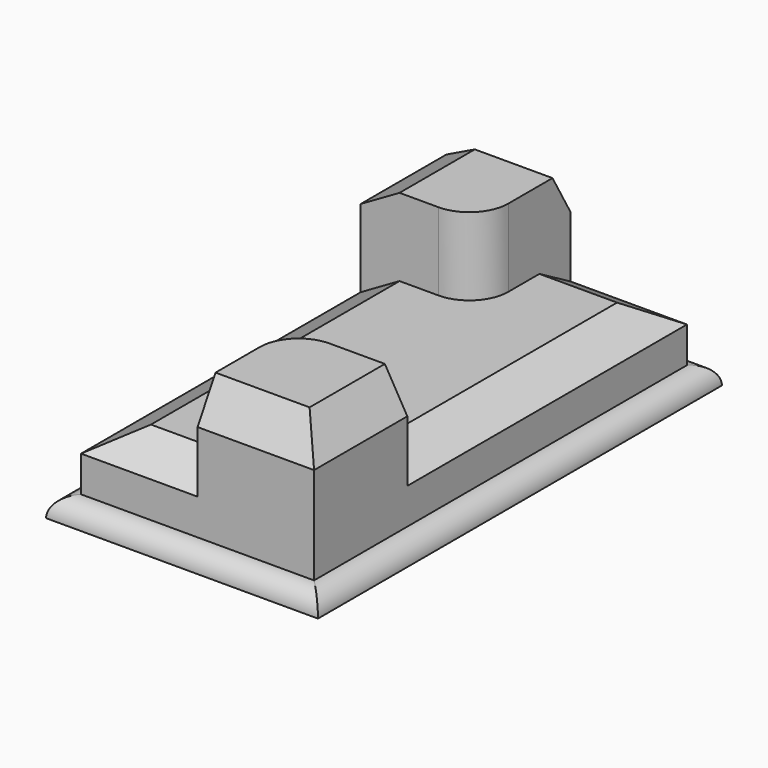
from build123d import *

# Parameters (mm, degrees)
F1_DEPTH    = 50.8
F2_DEPTH    = 25.4
F0_W        = 88.9
F0_H        = 165.1
F3_DEPTH    = 6.35
F4_SIZE2    = 7.3323484187
F4_SIZE     = 12.7
F5_C1_SIZE2 = 7.3323484187
F5_C1_SIZE  = 12.7
F5_C2_SIZE2 = 7.3323484187
F5_C2_SIZE  = 12.7
F5_C3_SIZE2 = 12.7
F5_C3_SIZE  = 7.3323484187
F5_C4_SIZE2 = 7.3323484187
F5_C4_SIZE  = 12.7
F6_R        = 6.34999


# Not quite as in the source:
# - a fillet or chamfer is up to 0.001 mm smaller than in the source, because OpenCascade refuses the exact size


with BuildPart() as f1:
    # F0 (on Top) → F1 (new body)
    with BuildSketch(Plane.XY):
        with BuildLine():
            Line((-19.9555572391, -85.2174787462), (-19.9555572391, -47.1174787462))
            Line((-19.9555572391, -47.1174787462), (-45.3555572391, -47.1174787462))
            ThreePointArc((-45.3555572391, -47.1174787462), (-54.3358133601, -50.8372226251), (-58.0555572391, -59.8174787462))
            Line((-58.0555572391, -59.8174787462), (-58.0555572391, -85.2174787462))
            Line((-58.0555572391, -85.2174787462), (-19.9555572391, -85.2174787462))
        make_face()
    extrude(amount=F1_DEPTH)



with BuildPart() as f1b:
    # F0 (on Top) → F1, piece 2 (new body)
    with BuildSketch(Plane.XY):
        with BuildLine():
            Line((-58.0555572391, 67.1825212538), (-96.1555572391, 67.1825212538))
            Line((-96.1555572391, 67.1825212538), (-96.1555572391, 29.0825212538))
            Line((-96.1555572391, 29.0825212538), (-70.7555572391, 29.0825212538))
            ThreePointArc((-70.7555572391, 29.0825212538), (-61.775301118, 32.8022651328), (-58.0555572391, 41.7825212538))
            Line((-58.0555572391, 41.7825212538), (-58.0555572391, 67.1825212538))
        make_face()
    extrude(amount=F1_DEPTH)


with BuildPart() as f1_1:
    add(f1.part)

    add(f1b.part)  # F2 merges F1b
    # F0 (on Top) → F2 (join)
    with BuildSketch(Plane.XY):
        with BuildLine():
            Line((-19.9555572391, 67.1825212538), (-58.0555572391, 67.1825212538))
            Line((-58.0555572391, 67.1825212538), (-58.0555572391, 41.7825212538))
            ThreePointArc((-58.0555572391, 41.7825212538), (-61.775301118, 32.8022651328), (-70.7555572391, 29.0825212538))
            Line((-70.7555572391, 29.0825212538), (-96.1555572391, 29.0825212538))
            Line((-96.1555572391, 29.0825212538), (-96.1555572391, -85.2174787462))
            Line((-96.1555572391, -85.2174787462), (-58.0555572391, -85.2174787462))
            Line((-58.0555572391, -85.2174787462), (-58.0555572391, -59.8174787462))
            ThreePointArc((-58.0555572391, -59.8174787462), (-54.3358133601, -50.8372226251), (-45.3555572391, -47.1174787462))
            Line((-45.3555572391, -47.1174787462), (-19.9555572391, -47.1174787462))
            Line((-19.9555572391, -47.1174787462), (-19.9555572391, 67.1825212538))
        make_face()
    extrude(amount=F2_DEPTH)

    # F0 (on Top) → F3 (join)
    with BuildSketch(Plane.XY):
        with Locations((-58.0555572391, -9.0174787462)):
            Rectangle(F0_W, F0_H)
        Polygon((-96.1555572391, 29.0825212538), (-96.1555572391, 67.1825212538), (-58.0555572391, 67.1825212538), (-19.9555572391, 67.1825212538), (-19.9555572391, -47.1174787462), (-19.9555572391, -85.2174787462), (-58.0555572391, -85.2174787462), (-96.1555572391, -85.2174787462), align=None, mode=Mode.SUBTRACT)
    extrude(amount=F3_DEPTH)

    # F4
    f4_edges = [f1_1.edges().sort_by_distance(p)[0] for p in [
        (-96.155557, -28.067479, 25.4),
        (-77.105557, -85.217479, 25.4),
        (-19.955557, 10.032521, 25.4),
        (-39.005557, 67.182521, 25.4),
    ]]
    f4_side = f1_1.faces().sort_by_distance((-58.055557, -9.017479, 25.4))[0]
    chamfer(f4_edges, length=F4_SIZE, length2=F4_SIZE2, reference=f4_side)

    # F5: chamfer of 12.7 x 7.3323484187 on 4 edges, made by hand

    # F5_c1
    f5_c1_edges = [f1_1.edges().sort_by_distance(p)[0] for p in [
        (-77.1055572391, 67.1825212538, 50.8),
    ]]
    f5_c1_side = f1_1.faces().sort_by_distance((-77.1055572391, 67.1825212538, 50.6533530316))[0]
    chamfer(f5_c1_edges, length=F5_C1_SIZE, length2=F5_C1_SIZE2, reference=f5_c1_side)

    # F5_c2
    f5_c2_edges = [f1_1.edges().sort_by_distance(p)[0] for p in [
        (-19.9555572391, -66.1674787462, 50.8),
    ]]
    f5_c2_side = f1_1.faces().sort_by_distance((-19.9555572391, -66.1674787462, 50.6533530316))[0]
    chamfer(f5_c2_edges, length=F5_C2_SIZE, length2=F5_C2_SIZE2, reference=f5_c2_side)

    # F5_c3
    f5_c3_edges = [f1_1.edges().sort_by_distance(p)[0] for p in [
        (-96.1555572391, 44.4663470445, 50.8),
    ]]
    f5_c3_side = f1_1.faces().sort_by_distance((-96.1555572391, 44.4663470445, 50.6533530316))[0]
    chamfer(f5_c3_edges, length=F5_C3_SIZE, length2=F5_C3_SIZE2, reference=f5_c3_side)

    # F5_c4
    f5_c4_edges = [f1_1.edges().sort_by_distance(p)[0] for p in [
        (-42.6717314484, -85.2174787462, 50.8),
    ]]
    f5_c4_side = f1_1.faces().sort_by_distance((-42.6717314484, -85.2174787462, 50.6533530316))[0]
    chamfer(f5_c4_edges, length=F5_C4_SIZE, length2=F5_C4_SIZE2, reference=f5_c4_side)

    # F6 (radius 6.35 in the source; OpenCascade refuses exactly that, so slightly less here)
    f6_edges = [f1_1.edges().sort_by_distance(p)[0] for p in [
        (-58.055557, -91.567479, 6.35),
        (-13.605557, -9.017479, 6.35),
        (-102.505557, -9.017479, 6.35),
        (-58.055557, 73.532521, 6.35),
    ]]
    fillet(f6_edges, radius=F6_R)


solid = f1_1.part
